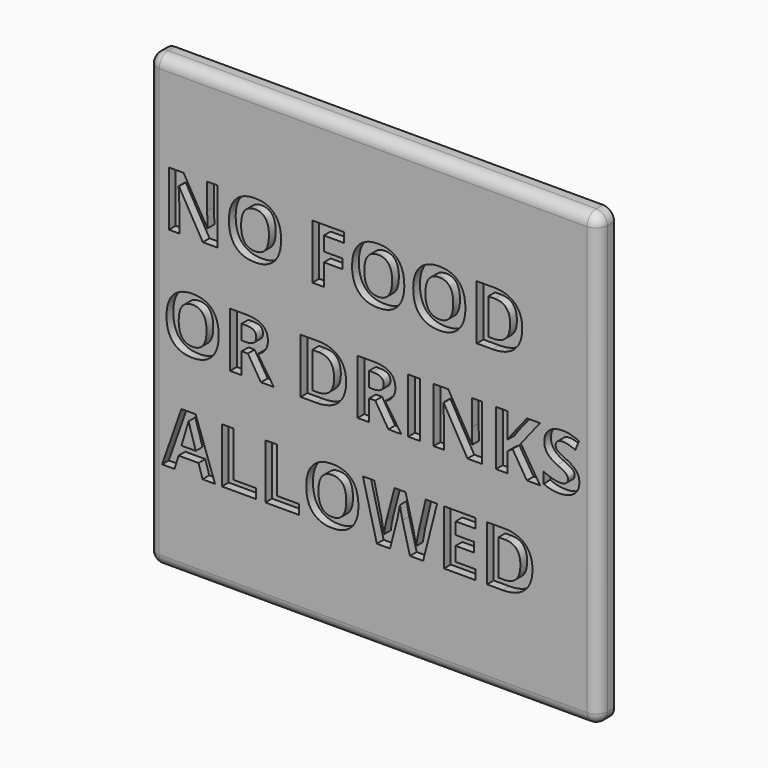
from build123d import *

# Parameters (mm, degrees)
F0_W         = 203.2
F0_H         = 203.2
F1_DEPTH     = 8.89
F2_TEXT_SIZE = 34.6324281332
F3_DEPTH     = 3.81
F4_R         = 5.08
F5_T1_DEPTH  = 16.51
F5_S5_W      = 5.08
F5_S5_H      = 5.08
F5_T6_DEPTH  = 5.08
F6_T1_DEPTH  = 16.51
F6_S5_W      = 5.08
F6_S5_H      = 5.08
F6_T6_DEPTH  = 5.08
F6_S11_W     = 5.08
F6_S11_H     = 5.08
F6_T12_DEPTH = 5.08
F6_S17_W     = 5.08
F6_S17_H     = 5.08
F6_T18_DEPTH = 5.08


# Not quite as in the source:
# - a fillet or chamfer that OpenCascade refuses, or shapes differently, is made with other operations: its cross-section is extruded or revolved along the edge and cut away or added
# - Text() gives the source's letters only with a copy of the font that has no kerning and outlines rounded to 1/6400 em; it was checked with that copy


with BuildPart() as f1:
    # F0 (on Front) → F1 (new body)
    with BuildSketch(Plane.XZ):
        Rectangle(F0_W, F0_H)
    extrude(amount=F1_DEPTH)

    # F2 (on face) → F3 (cut)
    with BuildSketch(Plane.XZ.offset(8.89)):
        with Locations((-95.25, 33.9699364108)):
            Text('NO FOOD', F2_TEXT_SIZE, font='Open Sans', font_style=FontStyle.BOLD, text_align=(TextAlign.LEFT, TextAlign.BOTTOM))
        with Locations((-95.25, -13.1301658503)):
            Text('OR DRINKS', F2_TEXT_SIZE, font='Open Sans', font_style=FontStyle.BOLD, text_align=(TextAlign.LEFT, TextAlign.BOTTOM))
        with Locations((-95.25, -60.2302681114)):
            Text('ALLOWED', F2_TEXT_SIZE, font='Open Sans', font_style=FontStyle.BOLD, text_align=(TextAlign.LEFT, TextAlign.BOTTOM))
    extrude(amount=-F3_DEPTH, mode=Mode.SUBTRACT)

    # F4
    f4_edges = [f1.edges().sort_by_distance(p)[0] for p in [
        (0, -8.89, 101.6),
        (-101.6, -8.89, 0),
        (0, -8.89, -101.6),
        (101.6, -8.89, 0),
    ]]
    fillet(f4_edges, radius=F4_R)

    # F5: fillet of radius 5.08 on 1 edges, made by hand

    # F5_s2 → F5_t1 (cut)
    with BuildSketch(Plane.XZ.offset(-12.7)):
        with BuildLine():
            ThreePointArc((101.6, 96.52), (100.1121024484, 100.1121024484), (96.52, 101.6))
            Line((96.52, 101.6), (101.6, 101.6))
            Line((101.6, 101.6), (101.6, 96.52))
        make_face()
    extrude(amount=F5_T1_DEPTH, mode=Mode.SUBTRACT)


with BuildPart() as f5_tool4:
    # F5_s5 → F5_t6 (new body)
    with BuildSketch(Plane.YZ.offset(96.52)):
        with Locations((-6.35, 99.06)):
            Rectangle(F5_S5_W, F5_S5_H)
    extrude(amount=F5_T6_DEPTH)

    # F5_s7 → F5_t8 (revolve, cut)
    with BuildSketch(Plane(origin=(96.52, -3.81, 96.52), x_dir=(0, 0.7071067812, -0.7071067812), z_dir=(0, -0.7071067812, -0.7071067812))):
        with BuildLine():
            ThreePointArc((0, -5.08), (5.08, 0), (0, 5.08))
            Line((0, 5.08), (0, -5.08))
        make_face()
    revolve(axis=Axis((96.52, -3.81, 96.52), (1, 0, 0)), mode=Mode.SUBTRACT)


with BuildPart() as f1_1:
    add(f1.part)

    # F5_t3: cut F5_tool4
    add(f5_tool4.part, mode=Mode.SUBTRACT)

    # F6: fillet of radius 5.08 on 3 edges, made by hand

    # F6_s2 → F6_t1 (cut)
    with BuildSketch(Plane.XZ.offset(-12.7)):
        with BuildLine():
            ThreePointArc((101.6, -96.52), (100.1121024484, -100.1121024484), (96.52, -101.6))
            Line((96.52, -101.6), (101.6, -101.6))
            Line((101.6, -101.6), (101.6, -96.52))
        make_face()
        with BuildLine():
            ThreePointArc((-96.52, -101.6), (-100.1121024484, -100.1121024484), (-101.6, -96.52))
            Line((-101.6, -96.52), (-101.6, -101.6))
            Line((-101.6, -101.6), (-96.52, -101.6))
        make_face()
        with BuildLine():
            ThreePointArc((-101.6, 96.52), (-100.1121024484, 100.1121024484), (-96.52, 101.6))
            Line((-96.52, 101.6), (-101.6, 101.6))
            Line((-101.6, 101.6), (-101.6, 96.52))
        make_face()
    extrude(amount=F6_T1_DEPTH, mode=Mode.SUBTRACT)


with BuildPart() as f6_tool4:
    # F6_s5 → F6_t6 (new body)
    with BuildSketch(Plane.YZ.offset(-96.52)):
        with Locations((-6.35, 99.06)):
            Rectangle(F6_S5_W, F6_S5_H)
    extrude(amount=-F6_T6_DEPTH)

    # F6_s7 → F6_t8 (revolve, cut)
    with BuildSketch(Plane(origin=(-96.52, -3.81, 96.52), x_dir=(0, 0.7071067812, -0.7071067812), z_dir=(0, 0.7071067812, 0.7071067812))):
        with BuildLine():
            ThreePointArc((0, -5.08), (5.08, 0), (0, 5.08))
            Line((0, 5.08), (0, -5.08))
        make_face()
    revolve(axis=Axis((-96.52, -3.81, 96.52), (-1, 0, 0)), mode=Mode.SUBTRACT)


with BuildPart() as f1_2:
    add(f1_1.part)

    # F6_t3: cut F6_tool4
    add(f6_tool4.part, mode=Mode.SUBTRACT)


with BuildPart() as f6_tool10:
    # F6_s11 → F6_t12 (new body)
    with BuildSketch(Plane.XY.offset(-96.52)):
        with Locations((-99.06, -6.35)):
            Rectangle(F6_S11_W, F6_S11_H)
    extrude(amount=-F6_T12_DEPTH)

    # F6_s13 → F6_t14 (revolve, cut)
    with BuildSketch(Plane(origin=(-96.52, -3.81, -96.52), x_dir=(0.7071067812, 0.7071067812, 0), z_dir=(-0.7071067812, 0.7071067812, 0))):
        with BuildLine():
            ThreePointArc((0, -5.08), (5.08, 0), (0, 5.08))
            Line((0, 5.08), (0, -5.08))
        make_face()
    revolve(axis=Axis((-96.52, -3.81, -96.52), (0, 0, -1)), mode=Mode.SUBTRACT)


with BuildPart() as f1_3:
    add(f1_2.part)

    # F6_t9: cut F6_tool10
    add(f6_tool10.part, mode=Mode.SUBTRACT)


with BuildPart() as f6_tool16:
    # F6_s17 → F6_t18 (new body)
    with BuildSketch(Plane.YZ.offset(96.52)):
        with Locations((-6.35, -99.06)):
            Rectangle(F6_S17_W, F6_S17_H)
    extrude(amount=F6_T18_DEPTH)

    # F6_s19 → F6_t20 (revolve, cut)
    with BuildSketch(Plane(origin=(96.52, -3.81, -96.52), x_dir=(0, 0.7071067812, 0.7071067812), z_dir=(0, 0.7071067812, -0.7071067812))):
        with BuildLine():
            ThreePointArc((0, -5.08), (5.08, 0), (0, 5.08))
            Line((0, 5.08), (0, -5.08))
        make_face()
    revolve(axis=Axis((96.52, -3.81, -96.52), (1, 0, 0)), mode=Mode.SUBTRACT)


with BuildPart() as f1_4:
    add(f1_3.part)

    # F6_t15: cut F6_tool16
    add(f6_tool16.part, mode=Mode.SUBTRACT)


solid = f1_4.part
